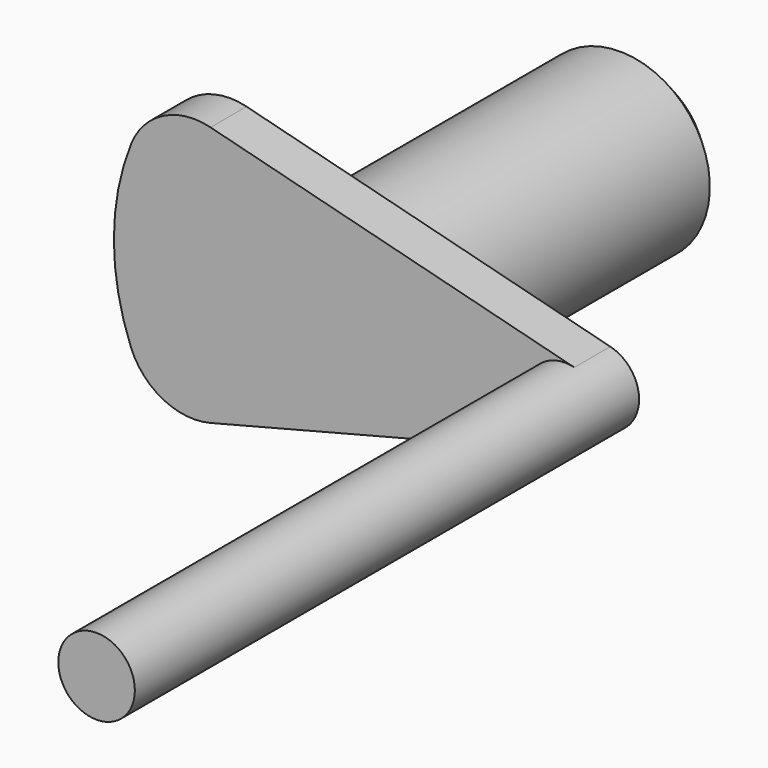
from build123d import *

# Parameters (mm, degrees)
F1_DEPTH = 2
F3_DEPTH = 26
F4_R     = 4
F5_DEPTH = 15
F6_SIZE  = 1


with BuildPart() as f1:
    # F0 (on Front) → F1 (new body)
    with BuildSketch(Plane.XZ):
        with BuildLine():
            ThreePointArc((10.7772780728, -1.6469869803), (11.6988240407, -1.0425715004), (12.0560490534, 0))
            ThreePointArc((12.0560490534, 0), (11.6988240407, 1.0425715004), (10.7772780728, 1.6469869803))
            Line((10.7772780728, 1.6469869803), (-5.3807416604, 5.7795192287))
            ThreePointArc((-5.3807416604, 5.7795192287), (-7.4835794739, 5.5473528625), (-8.9103223258, 3.9852283712))
            ThreePointArc((-8.9103223258, 3.9852283712), (-9.4830781383, 2.0290875977), (-9.6763123684, 0))
            ThreePointArc((-9.6763123684, 0), (-9.4830781383, -2.0290875977), (-8.9103223258, -3.9852283712))
            ThreePointArc((-8.9103223258, -3.9852283712), (-7.4835794739, -5.5473528625), (-5.3807416604, -5.7795192287))
            Line((-5.3807416604, -5.7795192287), (10.7772780728, -1.6469869803))
        make_face()
    extrude(amount=F1_DEPTH)

    # F2 (on face) → F3 (join)
    with BuildSketch(Plane.XZ.offset(2)):
        with BuildLine():
            ThreePointArc((10.7772780728, -1.6469869803), (11.6988240407, -1.0425715004), (12.0560490534, 0))
            ThreePointArc((12.0560490534, 0), (11.6988240407, 1.0425715004), (10.7772780728, 1.6469869803))
            ThreePointArc((10.7772780728, 1.6469869803), (8.6560490534, 0), (10.7772780728, -1.6469869803))
        make_face()
    extrude(amount=F3_DEPTH)

    # F4 (on face) → F5 (join)
    with BuildSketch(Plane(origin=(0, 0, 0), x_dir=(-1, 0, 0), z_dir=(0, 1, 0))):
        Circle(F4_R)
    extrude(amount=F5_DEPTH)

    # F6
    f6_edges = [f1.edges().sort_by_distance(p)[0] for p in [
        (4, 15, 0),
    ]]
    chamfer(f6_edges, length=F6_SIZE)


solid = f1.part
